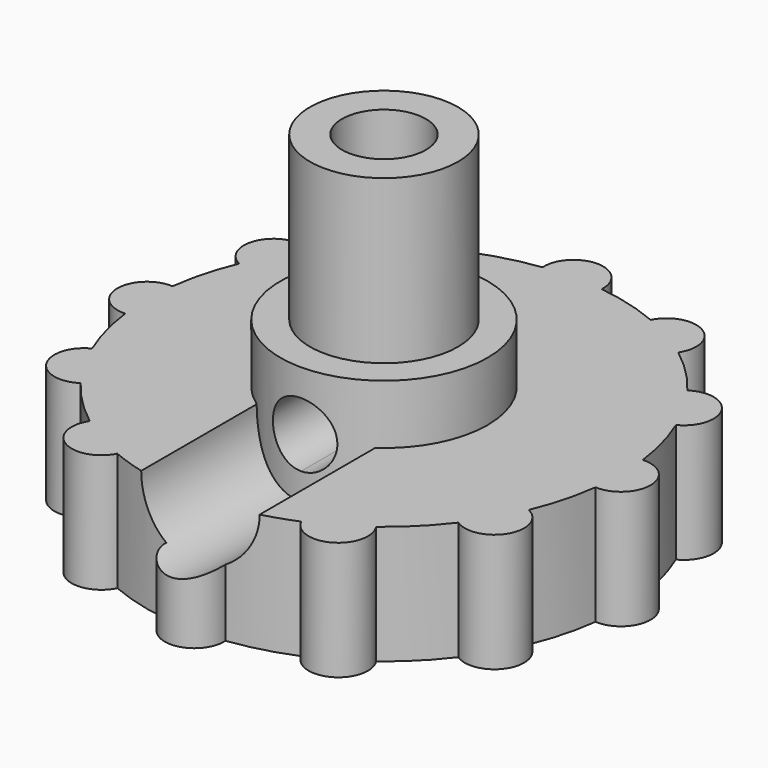
from build123d import *

# Parameters (mm, degrees)
F0_R           = 12.7
F1_DEPTH       = 6.35
F3_DEPTH       = 3.175
F4_R           = 5.55625
F5_DEPTH       = 3.175
F6_R           = 3.96875
F7_DEPTH       = 8.73125
F8_R           = 2.2479
F9_DEPTH       = 15.08125
F11_DEPTH      = 6.35
F12_COUNT      = 12
F12_ANGLE      = 330
F14_END_RADIUS = 5.55625
F14_REACH      = 18.1506366107
F17_END_RADIUS = 5.55625
F17_REACH      = 35.6755158286


with BuildPart() as f1:
    # F0 (on Top) → F1 (new body)
    with BuildSketch(Plane.XY):
        Circle(F0_R)
    extrude(amount=F1_DEPTH)

    # F2 (on face) → F3 (cut)
    with BuildSketch(Plane(origin=(0, 0, 0), x_dir=(1, 0, 0), z_dir=(0, 0, -1))):
        Polygon((2.2913588808, 3.96875), (-2.2913588808, 3.96875), (-4.5827177617, 0), (-2.2913588808, -3.96875), (2.2913588808, -3.96875), (4.5827177617, 0), align=None)
    extrude(amount=-F3_DEPTH, mode=Mode.SUBTRACT)

    # F4 (on face) → F5 (join)
    with BuildSketch(Plane.XY.offset(6.35)):
        Circle(F4_R)
    extrude(amount=F5_DEPTH)

    # F6 (on face) → F7 (join)
    with BuildSketch(Plane.XY.offset(9.525)):
        Circle(F6_R)
    extrude(amount=F7_DEPTH)

    # F8 (on face) → F9 (cut, through all)
    with BuildSketch(Plane(origin=(0, 0, 3.175), x_dir=(1, 0, 0), z_dir=(0, 0, -1))):
        Circle(F8_R)
    extrude(amount=-F9_DEPTH, mode=Mode.SUBTRACT)

    # F10 (on face) → F11 (join, through all)
    with BuildSketch(Plane(origin=(0, 0, 0), x_dir=(1, 0, 0), z_dir=(0, 0, -1))):
        with BuildLine():
            ThreePointArc((-1.5843963802, 12.60078125), (0, 12.7), (1.5843963802, 12.60078125))
            ThreePointArc((1.5843963802, 12.60078125), (0, 14.2875), (-1.5843963802, 12.60078125))
        make_face()
    f11 = extrude(amount=-F11_DEPTH)

    # F12: F11 ×12 about axis
    f12_axis = Axis((0, 0, 0), (0, 0, -1))
    for i in range(1, F12_COUNT):
        add(f11.rotate(f12_axis, i * F12_ANGLE / (F12_COUNT - 1)))

    f14_end = (Plane(origin=(0, 0, 7.9375), x_dir=(-1, 0, 0), z_dir=(0, 0, -1)) * Cylinder(F14_END_RADIUS, 124.9884067655, mode=Mode.PRIVATE)).faces().sort_by_distance((-5.55625, 0, 7.9375))[0]
    # F13 (on Front) → F14 (cut, up to the whole of a round face its end follows)
    with BuildSketch(Plane.XZ):
        with BuildLine():
            ThreePointArc((0, 8.0772), (-1.7272, 6.35), (0, 4.6228))
            Line((0, 4.6228), (0, 8.0772))
        make_face()
        with BuildLine():
            Line((0, 8.0772), (0, 4.6228))
            ThreePointArc((0, 4.6228), (1.2213148325, 5.1286851675), (1.7272, 6.35))
            ThreePointArc((1.7272, 6.35), (1.2213148325, 7.5713148325), (0, 8.0772))
        make_face()
    f14_long = extrude(amount=F14_REACH, mode=Mode.PRIVATE)
    add(split(f14_long, bisect_by=f14_end, keep=Keep.BOTTOM, mode=Mode.PRIVATE), mode=Mode.SUBTRACT)

    f17_end = (Plane(origin=(0, 0, 7.9375), x_dir=(-1, 0, 0), z_dir=(0, 0, -1)) * Cylinder(F17_END_RADIUS, 160.0381652835, mode=Mode.PRIVATE)).faces().sort_by_distance((-5.55625, 0, 7.9375))[0]
    # F16 (on offset) → F17 (cut, up to the whole of a round face its end follows)
    with BuildSketch(Plane.XZ.offset(14.2875)):
        with BuildLine():
            Line((3.175, 6.35), (-3.175, 6.35))
            ThreePointArc((-3.175, 6.35), (0, 3.175), (3.175, 6.35))
        make_face()
    f17_long = extrude(amount=-F17_REACH, mode=Mode.PRIVATE)
    add(split(f17_long, bisect_by=f17_end, keep=Keep.ALL, mode=Mode.PRIVATE).solids().sort_by_distance((0, -14.2875, 5.0024881485))[0], mode=Mode.SUBTRACT)


solid = f1.part
